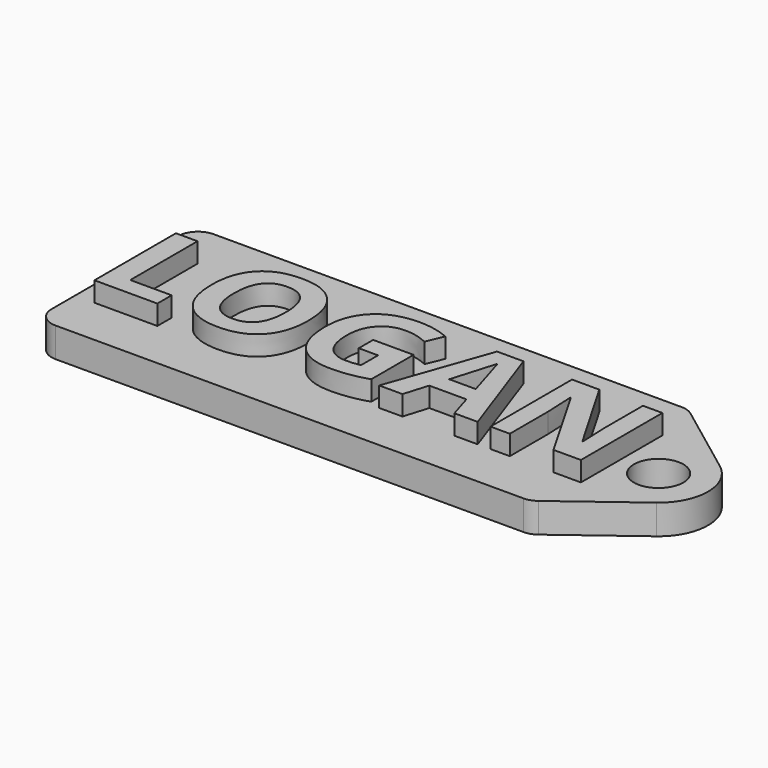
from build123d import *

# Parameters (mm, degrees)
F0_R         = 2.5
F1_DEPTH     = 3
F2_TEXT_SIZE = 14.4375003098
F3_DEPTH     = 2


# Not quite as in the source:
# - Text() gives the source's letters only with a copy of the font that has no kerning and outlines rounded to 1/6400 em; it was checked with that copy


with BuildPart() as f1:
    # F0 (on Top) → F1 (new body)
    with BuildSketch(Plane.XY):
        with BuildLine():
            Line((-23, -10), (24.3333333333, -10))
            ThreePointArc((24.3333333333, -10), (24.9657888654, -9.8973665961), (25.5333333333, -9.6))
            Line((25.5333333333, -9.6), (33, -4))
            ThreePointArc((33, -4), (34.472135955, -2.2360679775), (35, 0))
            ThreePointArc((35, 0), (34.472135955, 2.2360679775), (33, 4))
            Line((33, 4), (25.5333333333, 9.6))
            ThreePointArc((25.5333333333, 9.6), (24.9657888654, 9.8973665961), (24.3333333333, 10))
            Line((24.3333333333, 10), (-23, 10))
            ThreePointArc((-23, 10), (-24.4142135624, 9.4142135624), (-25, 8))
            Line((-25, 8), (-25, -8))
            ThreePointArc((-25, -8), (-24.4142135624, -9.4142135624), (-23, -10))
        make_face()
        with Locations((30, 0)):
            Circle(F0_R, mode=Mode.SUBTRACT)
    extrude(amount=F1_DEPTH)

    # F2 (on face) → F3 (join)
    with BuildSketch(Plane.XY.offset(3)):
        with Locations((-24.3337496649, -5.0400001928)):
            Text('LOGAN', F2_TEXT_SIZE, font='Open Sans', font_style=FontStyle.BOLD, text_align=(TextAlign.LEFT, TextAlign.BOTTOM))
    extrude(amount=F3_DEPTH)


solid = f1.part
